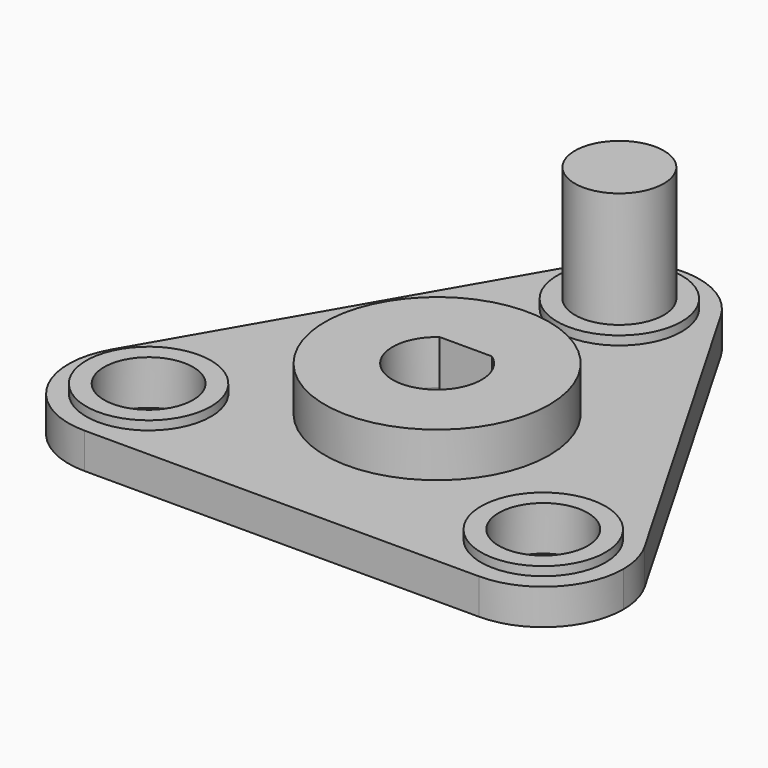
from build123d import *

# Parameters (mm, degrees)
F0_R     = 6.3000004034
F0_R_2   = 2.5
F1_DEPTH = 2
F2_R     = 6.3000004034
F3_DEPTH = 2.5
F4_R     = 3.5
F5_DEPTH = 0.5
F2_R_2   = 3.5
F2_R_3   = 2.5
F6_DEPTH = 0.5
F7_DEPTH = 9


# Not quite as in the source:
# - a feature names something its author has since deleted; it is built from what else it names


with BuildPart() as f1:
    # F0 (on Top) → F1 (new body)
    with BuildSketch(Plane.XY):
        with BuildLine():
            ThreePointArc((-14.9822403618, -4.1499987392), (-9.9204403472, -2.0533328369), (-6.5851262035, -6.3999990141))
            ThreePointArc((-6.5851262035, -6.3999990141), (-7.9031458296, -9.581979671), (-11.0851266037, -10.8999990141))
            Line((-11.0851266037, -10.8999990141), (11.0851230607, -10.9000009859))
            ThreePointArc((11.0851230607, -10.9000009859), (7.1880073569, -4.1499981658), (14.9822391266, -4.1499974067))
            Line((14.9822391266, -4.1499974067), (3.8971112321, 15.0500002429))
            ThreePointArc((3.8971112321, 15.0500002429), (4.3466632431, 13.9646860482), (4.4999970644, 12.8000004034))
            ThreePointArc((4.4999970644, 12.8000004034), (-1.1646868227, 8.4533357372), (-3.8971141748, 15.0499998963))
            Line((-3.8971141748, 15.0499998963), (-14.9822403618, -4.1499987392))
        make_face()
        Circle(F0_R, mode=Mode.SUBTRACT)
        Circle(F0_R)
        with BuildLine():
            ThreePointArc((1.4694631307, 2.0225424859), (2.2275163105, 1.1349762493), (2.5, 0))
            ThreePointArc((2.5, 0), (-1.1349762493, -2.2275163105), (-1.4694631307, 2.0225424859))
            ThreePointArc((-1.4694631307, 2.0225424859), (0, 2.5), (1.4694631307, 2.0225424859))
        make_face(mode=Mode.SUBTRACT)
        with BuildLine():
            ThreePointArc((14.9822391266, -4.1499974067), (7.1880073569, -4.1499981658), (11.0851230607, -10.9000009859))
            ThreePointArc((11.0851230607, -10.9000009859), (14.2671052289, -9.5819810652), (15.5851254326, -6.3999990141))
            ThreePointArc((15.5851254326, -6.3999990141), (15.4317914908, -5.2353124542), (14.9822391266, -4.1499974067))
        make_face()
        with Locations((11.0851234609, -6.3999990141)):
            Circle(F0_R_2, mode=Mode.SUBTRACT)
        with BuildLine():
            ThreePointArc((-11.0851266037, -10.8999990141), (-7.9031458296, -9.581979671), (-6.5851262035, -6.3999990141))
            ThreePointArc((-6.5851262035, -6.3999990141), (-9.9204403472, -2.0533328369), (-14.9822403618, -4.1499987392))
            ThreePointArc((-14.9822403618, -4.1499987392), (-14.9822406999, -8.6499987034), (-11.0851266037, -10.8999990141))
        make_face()
        with Locations((-11.0851262035, -6.3999990141)):
            Circle(F0_R_2, mode=Mode.SUBTRACT)
        with BuildLine():
            ThreePointArc((3.8971112321, 15.0500002429), (-1.5714e-06, 17.2999988391), (-3.8971141748, 15.0499998963))
            ThreePointArc((-3.8971141748, 15.0499998963), (-1.1646868227, 8.4533357372), (4.4999970644, 12.8000004034))
            ThreePointArc((4.4999970644, 12.8000004034), (4.3466632431, 13.9646860482), (3.8971112321, 15.0500002429))
        make_face()
        with Locations((-1.3713e-06, 12.8000004034)):
            Circle(F0_R_2, mode=Mode.SUBTRACT)
        with BuildLine():
            Line((-1.4694631307, 2.0225424859), (1.4694631307, 2.0225424859))
            ThreePointArc((1.4694631307, 2.0225424859), (0, 2.5), (-1.4694631307, 2.0225424859))
        make_face()
    extrude(amount=F1_DEPTH)

    # F2 (on face) → F3 (join)
    with BuildSketch(Plane.XY.offset(2)):
        Circle(F2_R)
        with BuildLine():
            Line((-1.4694631307, 2.0225424859), (1.4694631307, 2.0225424859))
            ThreePointArc((1.4694631307, 2.0225424859), (0, -2.5), (-1.4694631307, 2.0225424859))
        make_face(mode=Mode.SUBTRACT)
    extrude(amount=F3_DEPTH)

    # F2 (on face) → F6 (join)
    with BuildSketch(Plane.XY.offset(2)):
        with Locations((-1.3713e-06, 12.8000004034)):
            Circle(F2_R_2)
        with Locations((-1.3713e-06, 12.8000004034)):
            Circle(F2_R_3, mode=Mode.SUBTRACT)
        with Locations((-11.0851262035, -6.3999990141)):
            Circle(F2_R_2)
        with Locations((-11.0851262035, -6.3999990141)):
            Circle(F2_R_3, mode=Mode.SUBTRACT)
        with Locations((11.0851234609, -6.3999990141)):
            Circle(F2_R_2)
        with Locations((11.0851234609, -6.3999990141)):
            Circle(F2_R_3, mode=Mode.SUBTRACT)
    extrude(amount=F6_DEPTH)


with BuildPart() as f5:
    # F4 (on face) → F5 (new body)
    with BuildSketch(Plane(origin=(0, 0, 0), x_dir=(1, 0, 0), z_dir=(0, 0, -1))):
        Circle(F4_R)
        with BuildLine():
            ThreePointArc((-1.4694631307, -2.0225424859), (-1.1349762493, 2.2275163105), (2.5, 0))
            ThreePointArc((2.5, 0), (2.2275163105, -1.1349762493), (1.4694631307, -2.0225424859))
            ThreePointArc((1.4694631307, -2.0225424859), (0, -2.5), (-1.4694631307, -2.0225424859))
        make_face(mode=Mode.SUBTRACT)
    extrude(amount=F5_DEPTH)


with BuildPart() as f7:
    # F0 (on Top) → F7 (new body)
    with BuildSketch(Plane.XY):
        with Locations((-1.3713e-06, 12.8000004034)):
            Circle(F0_R_2)
    extrude(amount=F7_DEPTH)


solid = Compound([f1.part, f5.part, f7.part])
